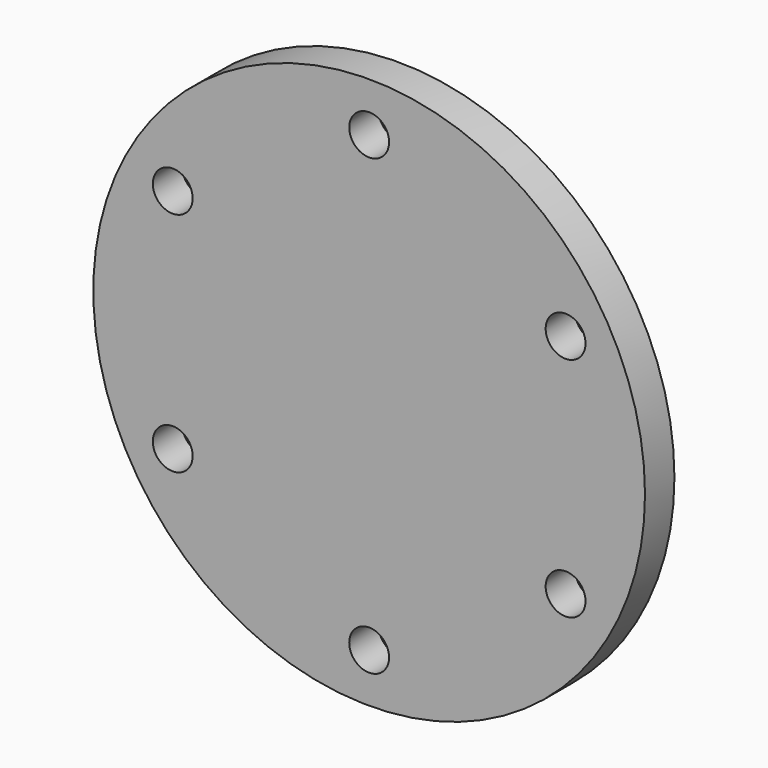
from build123d import *

# Parameters (mm, degrees)
F0_R            = 45
F1_DEPTH        = 3
F2_R            = 3.25
F3_DEPTH        = 25
F3_COPIES_COUNT = 6


# Not quite as in the source:
# - a pattern or mirror of a feature is missing from the dataset's text; its kind, count and spacing are read off the source's solid


with BuildPart() as f1:
    # F0 (on Front) → F1 (new body, symmetric)
    with BuildSketch(Plane.XZ):
        Circle(F0_R)
    extrude(amount=F1_DEPTH, both=True)

    # F2 (on face) → F3 (cut)
    with BuildSketch(Plane.XZ.offset(3)):
        with Locations((0, 37)):
            Circle(F2_R)
    f3 = extrude(amount=-F3_DEPTH, mode=Mode.SUBTRACT)

    # F3_copies: F3 ×6 about axis
    f3_copies_axis = Axis((0, 0, 0), (0, 1, 0))
    for i in range(1, F3_COPIES_COUNT):
        add(f3.rotate(f3_copies_axis, i * 360 / F3_COPIES_COUNT), mode=Mode.SUBTRACT)


solid = f1.part
